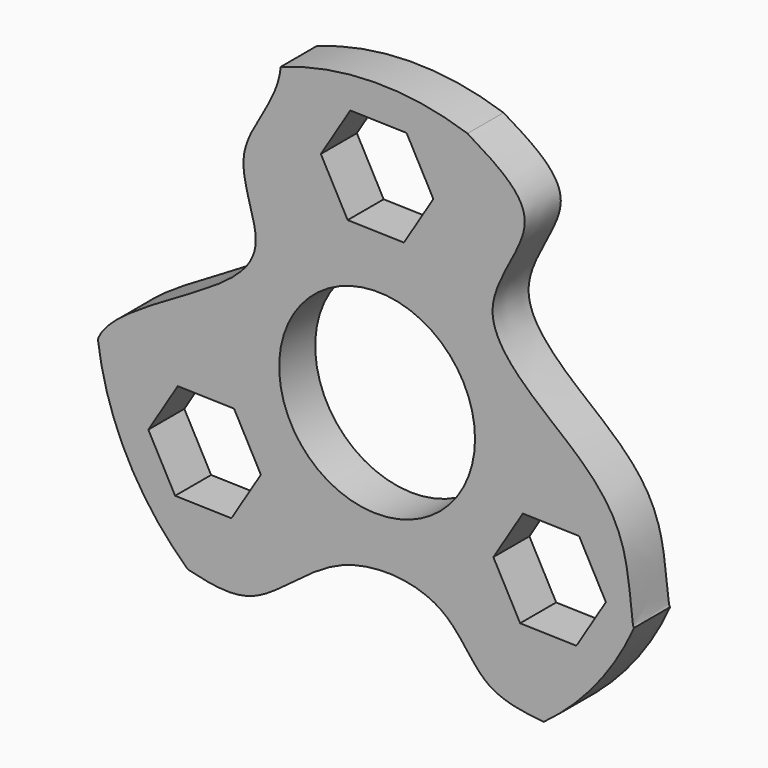
from build123d import *

# Parameters (mm, degrees)
F0_R            = 31.75
F0_R_2          = 11.049
F1_DEPTH        = 5.08
F3_DEPTH        = 25.4
F3_COPIES_COUNT = 3
F5_DEPTH        = 25.4
F7_DEPTH        = 25.4
F9_DEPTH        = 25.4


# Not quite as in the source:
# - a pattern or mirror of a feature is missing from the dataset's text; its kind, count and spacing are read off the source's solid


with BuildPart() as f1:
    # F0 (on Front) → F1 (new body)
    with BuildSketch(Plane.XZ):
        Circle(F0_R)
        Circle(F0_R_2, mode=Mode.SUBTRACT)
    extrude(amount=F1_DEPTH)

    # F2 (on face) → F3 (cut)
    with BuildSketch(Plane.XZ.offset(5.08)):
        Polygon((-6.3476239167, 22.6507535779), (-3.3242378834, 17.0667015641), (3.0233860333, 16.8930046675), (6.3476239167, 22.3033597847), (3.3242378834, 27.8874117986), (-3.0233860333, 28.0611086952), align=None)
    f3 = extrude(amount=-F3_DEPTH, mode=Mode.SUBTRACT)

    # F3_copies: F3 ×3 about axis
    f3_copies_axis = Axis((0, 0, 0), (0, 1, 0))
    for i in range(1, F3_COPIES_COUNT):
        add(f3.rotate(f3_copies_axis, i * 360 / F3_COPIES_COUNT), mode=Mode.SUBTRACT)

    # F4 (on face) → F5 (cut)
    with BuildSketch(Plane.XZ.offset(5.08)):
        with BuildLine():
            add(Edge.make_bspline(
                [(-31.5054908773, -3.9327527992), (-30.4212555796, -0.8719947567), (-18.3965247195, 4.8385711098), (-11.8105022121, 10.993768111), (-17.4986556453, 20.3648330822), (-11.1655893387, 26.0784288721), (-10.8861024487, 29.8254132155)],
                knots=[0.0786163527, 0.0786163527, 0.0786163527, 0.0786163527, 0.1981027466, 0.2848329917, 0.372394622, 0.4721628234, 0.4721628234, 0.4721628234, 0.4721628234], degree=3))
            ThreePointArc((-10.8861024487, 29.8254132155), (-27.0954837445, 16.5498417108), (-31.5054908773, -3.9327527992))
        make_face()
    extrude(amount=-F5_DEPTH, mode=Mode.SUBTRACT)

    # F6 (on face) → F7 (cut)
    with BuildSketch(Plane.XZ.offset(5.08)):
        with BuildLine():
            ThreePointArc((29.6280882801, -11.4122252373), (28.7525919392, 13.4666609364), (10.2008963701, 30.0666628219))
            add(Edge.make_bspline(
                [(10.2008963701, 30.0666628219), (13.429018895, 28.1108428572), (20.1420771241, 24.0166363798), (8.7498188411, 12.4166523035), (22.458442246, 2.918273975), (28.6476409792, -4.0514757745), (28.6704265074, -12.7852561952), (28.9986593393, -12.9282735322)],
                knots=[0, 0, 0, 0, 0.1765519892, 0.3676311546, 0.5795495459, 0.7701853291, 0.9256872831, 0.9256872831, 0.9256872831, 0.9256872831], degree=3))
            ThreePointArc((28.9986593393, -12.9282735322), (29.3231731693, -12.174317857), (29.6280882801, -11.4122252373))
        make_face()
    extrude(amount=-F7_DEPTH, mode=Mode.SUBTRACT)

    # F8 (on face) → F9 (cut)
    with BuildSketch(Plane.XZ.offset(5.08)):
        with BuildLine():
            add(Edge.make_bspline(
                [(-21.3469993385, -23.502513041), (-18.8943370089, -24.0879360583), (-13.3304325416, -25.3988350394), (-5.0598365774, -15.6071883389), (8.0966892993, -16.52845193), (11.5579864589, -24.7912307542), (16.4422151236, -25.3359894242), (18.7933290203, -25.5904920691)],
                knots=[0, 0, 0, 0, 0.182404748, 0.413031056, 0.6388938435, 0.8258884978, 1, 1, 1, 1], degree=3))
            ThreePointArc((-21.3469993385, -23.502513041), (-1.6493095916, -31.7071329179), (18.7933290203, -25.5904920691))
        make_face()
    extrude(amount=-F9_DEPTH, mode=Mode.SUBTRACT)


solid = f1.part
